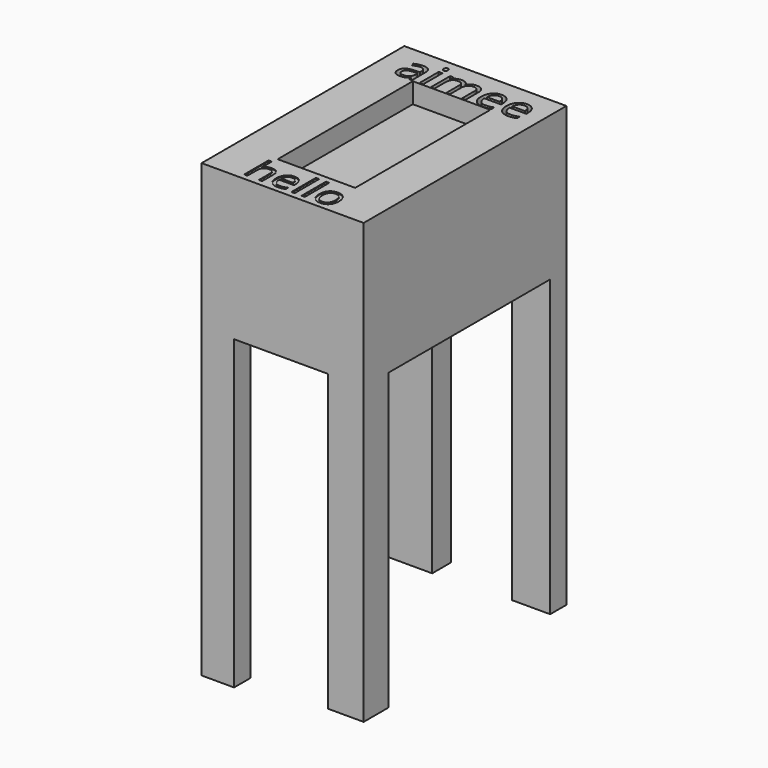
from build123d import *

# Parameters (mm, degrees)
F0_W          = 48.7189404666
F0_H          = 43.4386059642
F1_DEPTH      = 76.2
F2_T          = -12.7
F3_T          = -2.54
F4_W          = 9.7614619881
F4_H          = 6.2129488111
F5_DEPTH      = 92.202
F6_W          = 10.7381944545
F6_H          = 9.3778362393
F7_DEPTH      = 88.646
F8_W          = 14.0970274806
F8_H          = 7.1587194689
F8_W_2        = 11.5020358935
F8_H_2        = 6.0949302278
F9_DEPTH      = 56.388
F10_DEPTH     = 32.258
F11_W         = 11.6343349218
F11_H         = 12.360735786
F11_W_2       = 10.9820738435
F11_H_2       = 11.1142059481
F11_W_3       = 13.3966468275
F12_DEPTH     = 34.798
F13_W         = 48.7189404666
F13_H         = 76.2
F13_W_2       = 23.3189404666
F13_H_2       = 50.8
F14_DEPTH     = 25.4
F15_TEXT_SIZE = 12.099970546
F16_DEPTH     = 0.254
F18_TEXT_SIZE = 13.5623950175
F19_DEPTH     = 12.7


# Not quite as in the source:
# - Text() gives the source's letters only with a copy of the font that has no kerning and outlines rounded to 1/6400 em; it was checked with that copy


with BuildPart() as f1:
    # F0 (on Front) → F1 (new body)
    with BuildSketch(Plane.XZ):
        with Locations((-7.5227785856, 24.1580829024)):
            Rectangle(F0_W, F0_H)
    extrude(amount=F1_DEPTH)

    # F2
    f2_openings = [f1.faces().sort_by_distance(p)[0] for p in [
        (-7.522779, -38.1, 45.877386),
    ]]
    offset(amount=F2_T, openings=f2_openings)

    # F3
    f3_openings = [f1.faces().sort_by_distance(p)[0] for p in [
        (-7.522779, -76.2, 24.158083),
        (16.836692, -38.1, 24.158083),
        (-31.882249, -38.1, 24.158083),
    ]]
    offset(amount=F3_T, openings=f3_openings, kind=Kind.INTERSECTION)

    # F4 (on face) → F5 (join)
    with BuildSketch(Plane(origin=(0, 0, 2.4387799203), x_dir=(1, 0, 0), z_dir=(0, 0, -1))):
        with Locations((-27.0015178248, 73.0935255945)):
            Rectangle(F4_W, F4_H)
    extrude(amount=F5_DEPTH)

    # F6 (on face) → F7 (join)
    with BuildSketch(Plane(origin=(0, 0, 2.4387799203), x_dir=(1, 0, 0), z_dir=(0, 0, -1))):
        with Locations((11.4675944205, 71.5110818803)):
            Rectangle(F6_W, F6_H)
    extrude(amount=F7_DEPTH)

    # F8 (on face) → F9 (join)
    with BuildSketch(Plane(origin=(0, 0, 2.4387799203), x_dir=(1, 0, 0), z_dir=(0, 0, -1))):
        with Locations((-24.8337350786, 3.5793597344)):
            Rectangle(F8_W, F8_H)
        with Locations((11.085673701, 3.0474651139)):
            Rectangle(F8_W_2, F8_H_2)
    extrude(amount=F9_DEPTH)

    # F10 (add, through all): faces of the model
    f10_faces = [f1.faces().sort_by_distance(p)[0] for p in [
        (-24.8337350786, -3.5793597344, -53.9492200797),
        (11.085673701, -3.0474651139, -53.9492200797),
    ]]
    extrude(f10_faces, amount=F10_DEPTH)

    # F11 (on face) → F12 (join)
    with BuildSketch(Plane.XY.offset(4.9787799203)):
        with Locations((11.0195241868, -70.019632107)):
            Rectangle(F11_W, F11_H)
        with Locations((11.345654726, -8.0971029741)):
            Rectangle(F11_W_2, F11_H_2)
        Polygon((-18.4856019914, -76.2), (5.2023567259, -76.2), (5.2023567259, -63.839264214), (16.8366916478, -63.839264214), (16.8366916478, -13.6542059481), (5.8546178043, -13.6542059481), (5.8546178043, -2.54), (-31.8822488189, -2.54), (-31.8822488189, -63.839264214), (-18.4856019914, -63.839264214), align=None)
        with Locations((-25.1839254051, -70.019632107)):
            Rectangle(F11_W_3, F11_H)
    extrude(amount=F12_DEPTH)

    # F13 (on face) → F14 (join)
    with BuildSketch(Plane.XY.offset(45.8773858845)):
        with Locations((-7.5227785856, -38.1)):
            Rectangle(F13_W, F13_H)
        with Locations((-7.5227785856, -38.1)):
            Rectangle(F13_W_2, F13_H_2, mode=Mode.SUBTRACT)
    extrude(amount=-F14_DEPTH)

    # F15 (on face) → F16 (cut)
    with BuildSketch(Plane.XY.offset(45.8773858845)):
        with Locations((-21.504347038, -74.5000466704)):
            Text('hello', F15_TEXT_SIZE, font='Open Sans', text_align=(TextAlign.LEFT, TextAlign.BOTTOM))
    extrude(amount=-F16_DEPTH, mode=Mode.SUBTRACT)

    # F18 (on face) → F19 (cut)
    with BuildSketch(Plane.XY.offset(45.8773858845)):
        with Locations((-26.0974457487, -12.4504482374)):
            Text('aimee', F18_TEXT_SIZE, font='Open Sans', text_align=(TextAlign.LEFT, TextAlign.BOTTOM))
    extrude(amount=-F19_DEPTH, mode=Mode.SUBTRACT)


solid = f1.part
